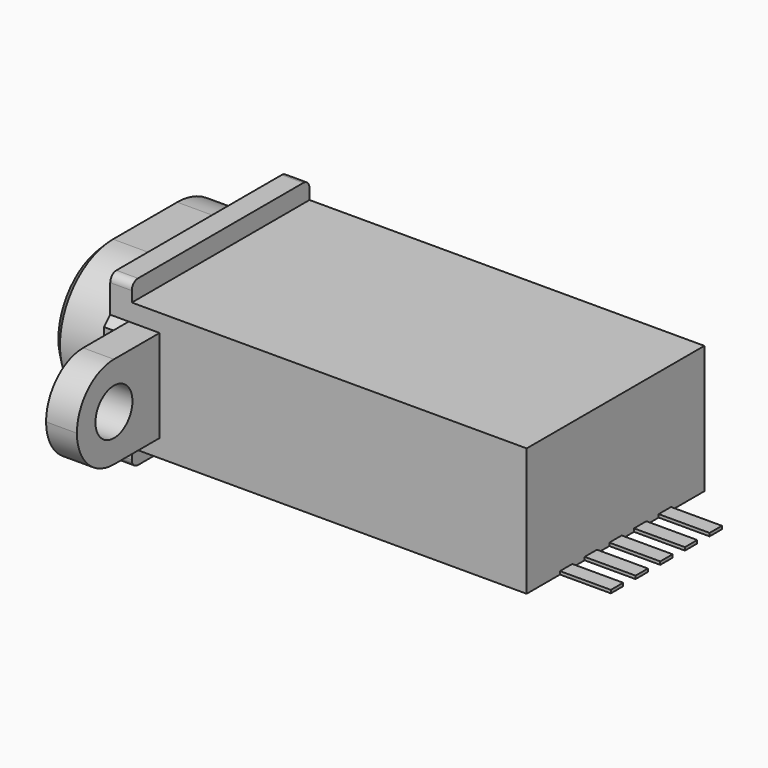
from build123d import *

# Parameters (mm, degrees)
F0_W      = 12.8
F0_H      = 7.2
F1_DEPTH  = 4.15
F2_W      = 0.25
F2_H      = 2.5
F2_W_2    = 7.2
F3_DEPTH  = 0.7
F4_R      = 1.5
F5_DEPTH  = 2
F6_SIZE   = 0.25
F7_W      = 1
F7_H      = 3
F8_DEPTH  = 3.35
F9_R      = 1.49999
F10_R     = 0.75
F11_DEPTH = 25
F12_R     = 0.5
F13_DEPTH = 0.5
F14_W     = 0.5
F14_H     = 0.1
F15_DEPTH = 14.45


# Not quite as in the source:
# - a fillet or chamfer is up to 0.001 mm smaller than in the source, because OpenCascade refuses the exact size


with BuildPart() as f1:
    # F0 (on Top) → F1 (new body)
    with BuildSketch(Plane.XY):
        with Locations((6.4, 0)):
            Rectangle(F0_W, F0_H)
    extrude(amount=F1_DEPTH)

    # F2 (on face) → F3 (join)
    with BuildSketch(Plane(origin=(0, 0, 0), x_dir=(0, -1, 0), z_dir=(-1, 0, 0))):
        with BuildLine():
            Line((3.35, 4.74), (-3.35, 4.74))
            ThreePointArc((-3.35, 4.74), (-3.5267766953, 4.6667766953), (-3.6, 4.49))
            Line((-3.6, 4.49), (-3.6, 3.575))
            Line((-3.6, 3.575), (-3.6, 3.325))
            Line((-3.6, 3.325), (3.6, 3.325))
            Line((3.6, 3.325), (3.6, 3.575))
            Line((3.6, 3.575), (3.6, 4.49))
            ThreePointArc((3.6, 4.49), (3.5267766953, 4.6667766953), (3.35, 4.74))
        make_face()
        Polygon((-3.6, 3.325), (-3.6, 3.575), (-3.85, 3.325), align=None)
        Polygon((3.85, 3.325), (3.6, 3.575), (3.6, 3.325), align=None)
        with Locations((-3.725, 2.075)):
            Rectangle(F2_W, F2_H)
        with Locations((3.725, 2.075)):
            Rectangle(F2_W, F2_H)
        with BuildLine():
            Line((3.6, 0.825), (-3.6, 0.825))
            Line((-3.6, 0.825), (-3.6, 0.575))
            Line((-3.6, 0.575), (-3.6, -0.34))
            ThreePointArc((-3.6, -0.34), (-3.5267766953, -0.5167766953), (-3.35, -0.59))
            Line((-3.35, -0.59), (3.35, -0.59))
            ThreePointArc((3.35, -0.59), (3.5267766953, -0.5167766953), (3.6, -0.34))
            Line((3.6, -0.34), (3.6, 0.575))
            Line((3.6, 0.575), (3.6, 0.825))
        make_face()
        Polygon((-3.6, 0.575), (-3.6, 0.825), (-3.85, 0.825), align=None)
        Polygon((3.85, 0.825), (3.6, 0.825), (3.6, 0.575), align=None)
        with Locations((0, 2.075)):
            Rectangle(F2_W_2, F2_H)
    extrude(amount=F3_DEPTH)

    # F4 (on face) → F5 (join)
    with BuildSketch(Plane(origin=(-0.7, 0, 0), x_dir=(0, -1, 0), z_dir=(-1, 0, 0))):
        with BuildLine():
            ThreePointArc((1.3, -0.075), (3.45, 2.075), (1.3, 4.225))
            Line((1.3, 4.225), (-1.3, 4.225))
            ThreePointArc((-1.3, 4.225), (-3.45, 2.075), (-1.3, -0.075))
            Line((-1.3, -0.075), (1.3, -0.075))
        make_face()
        with Locations((0, 2.075)):
            Circle(F4_R, mode=Mode.SUBTRACT)
    extrude(amount=F5_DEPTH)

    # F6
    f6_edges = [f1.edges().sort_by_distance(p)[0] for p in [
        (-2.7, 0, 4.225),
    ]]
    chamfer(f6_edges, length=F6_SIZE)

    # F7 (on face) → F8 (join)
    with BuildSketch(Plane.XZ.offset(3.6)):
        with Locations((0.4, 2.075)):
            Rectangle(F7_W, F7_H)
    extrude(amount=F8_DEPTH)

    # F9 (radius 1.5 in the source; OpenCascade refuses exactly that, so slightly less here)
    f9_edges = [f1.edges().sort_by_distance(p)[0] for p in [
        (0.4, -6.95, 3.575),
        (0.4, -6.95, 0.575),
    ]]
    fillet(f9_edges, radius=F9_R)

    # F10 (on face) → F11 (cut)
    with BuildSketch(Plane(origin=(-0.1, 0, 0), x_dir=(0, -1, 0), z_dir=(-1, 0, 0))):
        with Locations((5.45, 2.075)):
            Circle(F10_R)
    extrude(amount=-F11_DEPTH, mode=Mode.SUBTRACT)

    # F12 (on face) → F13 (join)
    with BuildSketch(Plane(origin=(0, 0, 0), x_dir=(1, 0, 0), z_dir=(0, 0, -1))):
        with Locations((2.3, 0)):
            Circle(F12_R)
        with Locations((7.3, 0)):
            Circle(F12_R)
    extrude(amount=F13_DEPTH)

    # F14 (on face) → F15 (join)
    with BuildSketch(Plane.YZ):
        with Locations((0, 0.05)):
            Rectangle(F14_W, F14_H)
        with Locations((1, 0.05)):
            Rectangle(F14_W, F14_H)
        with Locations((2, 0.05)):
            Rectangle(F14_W, F14_H)
        with Locations((-1, 0.05)):
            Rectangle(F14_W, F14_H)
        with Locations((-2, 0.05)):
            Rectangle(F14_W, F14_H)
    extrude(amount=F15_DEPTH)


solid = f1.part
